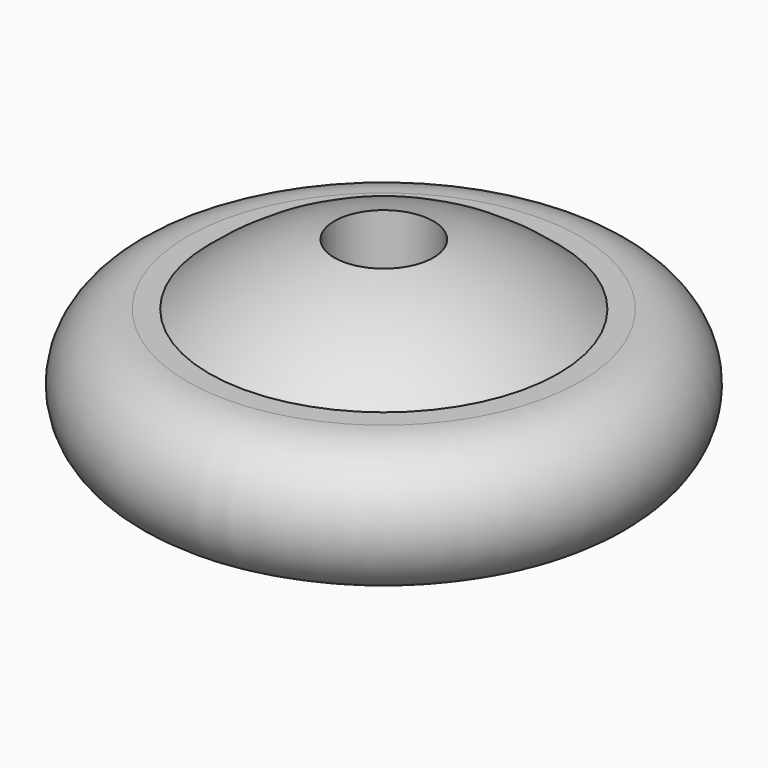
from build123d import *

# Parameters (mm, degrees)
F2_R          = 1.5
F3_DEPTH      = 3.999122753
F3_DEPTH_BACK = 4.0007233578


with BuildPart() as f1:
    # F0 (on Front) → F1 (revolve)
    with BuildSketch(Plane.XZ):
        with BuildLine():
            Line((-5.878140574, -1.9962841181), (-5.2933794143, -1.9964670559))
            ThreePointArc((-5.2933794143, -1.9964670559), (-2.8295976372, -3.4809950098), (0, -3.998122753))
            Line((0, -3.998122753), (0, 3.9997233578))
            ThreePointArc((0, 3.9997233578), (-2.8285996381, 3.4829729251), (-5.2917792545, 1.9994793797))
            Line((-5.2917792545, 1.9994793797), (-5.9530518044, 1.9994488908))
            ThreePointArc((-5.9530518044, 1.9994488908), (-7.9981910715, 0.0850437646), (-6.1231084445, -1.9962074819))
            Line((-6.1231084445, -1.9962074819), (-5.878140574, -1.9962841181))
        make_face()
        with BuildLine():
            ThreePointArc((-6.1231084445, -1.9962074819), (-6.0006256837, -1.9999999021), (-5.878140574, -1.9962841181))
            Line((-5.878140574, -1.9962841181), (-6.1231084445, -1.9962074819))
        make_face()
    revolve(axis=Axis((0, 0, 0.0008003024), (0, 0, -1)))

    # F2 (on Top) → F3 (cut, two sides)
    with BuildSketch(Plane.XY) as f3_sk:
        Circle(F2_R)
    extrude(amount=-F3_DEPTH, mode=Mode.SUBTRACT)
    extrude(f3_sk.sketch, amount=F3_DEPTH_BACK, mode=Mode.SUBTRACT)


solid = f1.part
